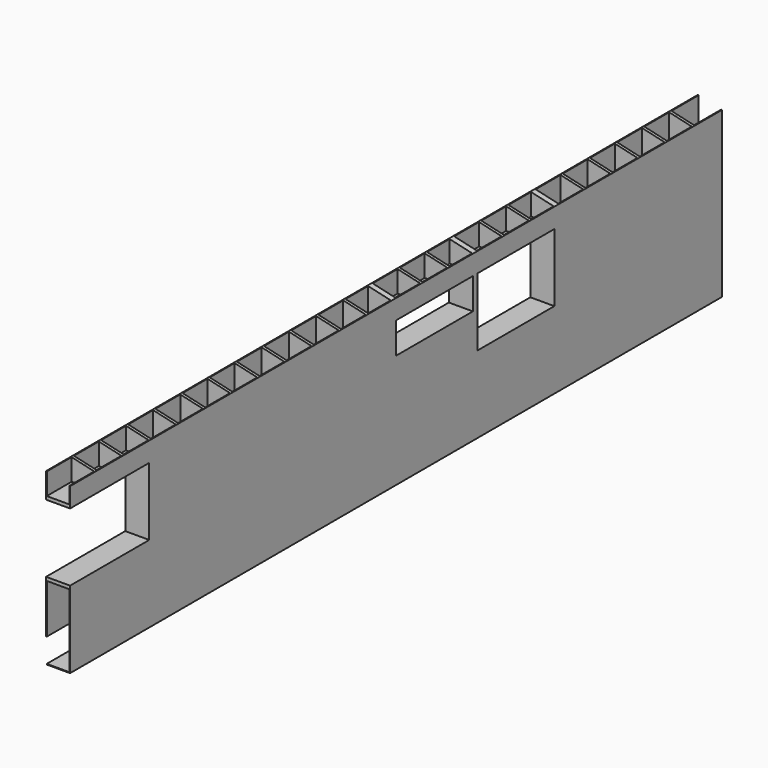
from build123d import *

# Parameters (mm, degrees)
F0_W     = 51
F0_H     = 590
F0_H_2   = 1290
F1_DEPTH = 400
F0_H_3   = 3200
F0_H_4   = 1940
F2_W     = 549
F2_H     = 590
F2_H_2   = 1290
F2_W_2   = 12600
F2_H_3   = 3200
F2_W_3   = 1698
F2_H_4   = 1200
F2_H_5   = 550
F3_DEPTH = 12
F4_W     = 12600
F4_H     = 2778
F4_W_2   = 1698
F4_H_2   = 1200
F4_H_3   = 550
F4_W_3   = 549
F4_H_4   = 590
F4_H_5   = 868
F5_DEPTH = 12
F7_DEPTH = 14400.001
F8_W     = 412
F8_H     = 14400
F9_DEPTH = 12


# Not quite as in the source:
# - a feature names something its author has since deleted; it is built from what else it names


with BuildPart() as f1:
    # F0 (on Right) → F1 (new body)
    with BuildSketch(Plane.YZ):
        with Locations((574.5, 2905)):
            Rectangle(F0_W, F0_H)
        with Locations((1174.5, 2905)):
            Rectangle(F0_W, F0_H)
        Polygon((1749, 2550), (1749, 1350), (1749, 1290), (1749, 0), (1800, 0), (1800, 3200), (1749, 3200), (1749, 2610), align=None)
        Polygon((0, 2610), (0, 2550), (1740, 2550), (1749, 2550), (1749, 2610), (1200, 2610), (1149, 2610), (600, 2610), (549, 2610), align=None)
        Polygon((0, 1350), (0, 1290), (549, 1290), (600, 1290), (1149, 1290), (1200, 1290), (1749, 1290), (1749, 1350), (1740, 1350), align=None)
        with Locations((1174.5, 645)):
            Rectangle(F0_W, F0_H_2)
        with Locations((574.5, 645)):
            Rectangle(F0_W, F0_H_2)
    extrude(amount=F1_DEPTH)



with BuildPart() as f1b:
    # F0 (on Right) → F1, piece 2 (new body)
    with BuildSketch(Plane.YZ):
        with Locations((2374.5, 1600)):
            Rectangle(F0_W, F0_H_3)
    extrude(amount=F1_DEPTH)


with BuildPart() as f1c:
    # F0 (on Right) → F1, piece 3 (new body)
    with BuildSketch(Plane.YZ):
        with Locations((2974.5, 1600)):
            Rectangle(F0_W, F0_H_3)
    extrude(amount=F1_DEPTH)


with BuildPart() as f1d:
    # F0 (on Right) → F1, piece 4 (new body)
    with BuildSketch(Plane.YZ):
        with Locations((3574.5, 1600)):
            Rectangle(F0_W, F0_H_3)
    extrude(amount=F1_DEPTH)


with BuildPart() as f1e:
    # F0 (on Right) → F1, piece 5 (new body)
    with BuildSketch(Plane.YZ):
        with Locations((4174.5, 1600)):
            Rectangle(F0_W, F0_H_3)
    extrude(amount=F1_DEPTH)


with BuildPart() as f1f:
    # F0 (on Right) → F1, piece 6 (new body)
    with BuildSketch(Plane.YZ):
        with Locations((4774.5, 1600)):
            Rectangle(F0_W, F0_H_3)
    extrude(amount=F1_DEPTH)


with BuildPart() as f1g:
    # F0 (on Right) → F1, piece 7 (new body)
    with BuildSketch(Plane.YZ):
        with Locations((5374.5, 1600)):
            Rectangle(F0_W, F0_H_3)
    extrude(amount=F1_DEPTH)


with BuildPart() as f1h:
    # F0 (on Right) → F1, piece 8 (new body)
    with BuildSketch(Plane.YZ):
        with Locations((5974.5, 1600)):
            Rectangle(F0_W, F0_H_3)
    extrude(amount=F1_DEPTH)


with BuildPart() as f1i:
    # F0 (on Right) → F1, piece 9 (new body)
    with BuildSketch(Plane.YZ):
        with Locations((6574.5, 1600)):
            Rectangle(F0_W, F0_H_3)
    extrude(amount=F1_DEPTH)


with BuildPart() as f1j:
    # F0 (on Right) → F1, piece 10 (new body)
    with BuildSketch(Plane.YZ):
        with Locations((7774.5, 2905)):
            Rectangle(F0_W, F0_H)
        with Locations((8374.5, 2905)):
            Rectangle(F0_W, F0_H)
        with Locations((9574.5, 2905)):
            Rectangle(F0_W, F0_H)
        with Locations((10174.5, 2905)):
            Rectangle(F0_W, F0_H)
        with Locations((10774.5, 1600)):
            Rectangle(F0_W, F0_H_3)
        Polygon((7149, 3200), (7149, 0), (7200, 0), (7200, 1940), (7749, 1940), (7800, 1940), (8349, 1940), (8400, 1940), (8898, 1940), (8898, 2000), (7200, 2000), (7200, 2550), (7200, 2610), (7200, 3200), align=None)
        with Locations((7774.5, 970)):
            Rectangle(F0_W, F0_H_4)
        Polygon((9549, 2610), (9000, 2610), (9000, 2550), (10698, 2550), (10698, 2610), (10200, 2610), (10149, 2610), (9600, 2610), align=None)
        Polygon((8949, 3200), (8949, 0), (9000, 0), (9000, 1290), (9000, 1350), (9000, 2550), (9000, 2610), (9000, 3200), align=None)
        with Locations((9574.5, 645)):
            Rectangle(F0_W, F0_H_2)
        with Locations((7123.5, 1600)):
            Rectangle(F0_W, F0_H_3)
        Polygon((7749, 2610), (7200, 2610), (7200, 2550), (8898, 2550), (8898, 2610), (8400, 2610), (8349, 2610), (7800, 2610), align=None)
        Polygon((9000, 1350), (9000, 1290), (9549, 1290), (9600, 1290), (10149, 1290), (10200, 1290), (10698, 1290), (10698, 1350), align=None)
        Polygon((8898, 2610), (8898, 2550), (8898, 2000), (8898, 1940), (8898, 0), (8949, 0), (8949, 3200), (8898, 3200), align=None)
        with Locations((10174.5, 645)):
            Rectangle(F0_W, F0_H_2)
        Polygon((10698, 2550), (10698, 1350), (10698, 1290), (10698, 0), (10749, 0), (10749, 3200), (10698, 3200), (10698, 2610), align=None)
        with Locations((8374.5, 970)):
            Rectangle(F0_W, F0_H_4)
    extrude(amount=F1_DEPTH)


with BuildPart() as f1k:
    # F0 (on Right) → F1, piece 11 (new body)
    with BuildSketch(Plane.YZ):
        with Locations((11374.5, 1600)):
            Rectangle(F0_W, F0_H_3)
    extrude(amount=F1_DEPTH)


with BuildPart() as f1l:
    # F0 (on Right) → F1, piece 12 (new body)
    with BuildSketch(Plane.YZ):
        with Locations((11974.5, 1600)):
            Rectangle(F0_W, F0_H_3)
    extrude(amount=F1_DEPTH)


with BuildPart() as f1m:
    # F0 (on Right) → F1, piece 13 (new body)
    with BuildSketch(Plane.YZ):
        with Locations((12574.5, 1600)):
            Rectangle(F0_W, F0_H_3)
    extrude(amount=F1_DEPTH)


with BuildPart() as f1n:
    # F0 (on Right) → F1, piece 14 (new body)
    with BuildSketch(Plane.YZ):
        with Locations((13174.5, 1600)):
            Rectangle(F0_W, F0_H_3)
    extrude(amount=F1_DEPTH)


with BuildPart() as f1o:
    # F0 (on Right) → F1, piece 15 (new body)
    with BuildSketch(Plane.YZ):
        with Locations((13774.5, 1600)):
            Rectangle(F0_W, F0_H_3)
    extrude(amount=F1_DEPTH)


with BuildPart() as f1_1:
    add(f1.part)

    add(f1b.part)  # F3 merges F1b

    add(f1c.part)  # F3 merges F1c

    add(f1d.part)  # F3 merges F1d

    add(f1e.part)  # F3 merges F1e

    add(f1f.part)  # F3 merges F1f

    add(f1g.part)  # F3 merges F1g

    add(f1h.part)  # F3 merges F1h

    add(f1i.part)  # F3 merges F1i

    add(f1j.part)  # F3 merges F1j

    add(f1k.part)  # F3 merges F1k

    add(f1l.part)  # F3 merges F1l

    add(f1m.part)  # F3 merges F1m

    add(f1n.part)  # F3 merges F1n

    add(f1o.part)  # F3 merges F1o
    # F2 (on face) → F3 (join)
    with BuildSketch(Plane.YZ.offset(400)):
        with Locations((274.5, 2905)):
            Rectangle(F2_W, F2_H)
        Polygon((600, 3200), (549, 3200), (549, 2610), (0, 2610), (0, 2550), (1749, 2550), (1749, 1350), (0, 1350), (0, 1290), (549, 1290), (549, 0), (600, 0), (600, 1290), (1149, 1290), (1149, 0), (1200, 0), (1200, 1290), (1749, 1290), (1749, 0), (1800, 0), (1800, 3200), (1749, 3200), (1749, 2610), (1200, 2610), (1200, 3200), (1149, 3200), (1149, 2610), (600, 2610), align=None)
        with Locations((874.5, 2905)):
            Rectangle(F2_W, F2_H)
        with Locations((1474.5, 2905)):
            Rectangle(F2_W, F2_H)
        with Locations((274.5, 645)):
            Rectangle(F2_W, F2_H_2)
        with Locations((8100, 1600)):
            Rectangle(F2_W_2, F2_H_3)
        with Locations((9849, 1950)):
            Rectangle(F2_W_3, F2_H_4, mode=Mode.SUBTRACT)
        with Locations((8049, 2275)):
            Rectangle(F2_W_3, F2_H_5, mode=Mode.SUBTRACT)
        with Locations((874.5, 645)):
            Rectangle(F2_W, F2_H_2)
        with Locations((1474.5, 645)):
            Rectangle(F2_W, F2_H_2)
    extrude(amount=F3_DEPTH)

    # F4 (on face) → F5 (join)
    with BuildSketch(Plane(origin=(0, 0, 0), x_dir=(0, -1, 0), z_dir=(-1, 0, 0))):
        with Locations((-8100, 1811)):
            Rectangle(F4_W, F4_H)
        with Locations((-9849, 1950)):
            Rectangle(F4_W_2, F4_H_2, mode=Mode.SUBTRACT)
        with Locations((-8049, 2275)):
            Rectangle(F4_W_2, F4_H_3, mode=Mode.SUBTRACT)
        Polygon((-1749, 3200), (-1800, 3200), (-1800, 422), (-1749, 422), (-1749, 1290), (-1200, 1290), (-1200, 422), (-1149, 422), (-1149, 1290), (-600, 1290), (-600, 422), (-549, 422), (-549, 1290), (0, 1290), (0, 1350), (-1749, 1350), (-1749, 2550), (0, 2550), (0, 2610), (-549, 2610), (-549, 3200), (-600, 3200), (-600, 2610), (-1149, 2610), (-1149, 3200), (-1200, 3200), (-1200, 2610), (-1749, 2610), align=None)
        with Locations((-1474.5, 2905)):
            Rectangle(F4_W_3, F4_H_4)
        with Locations((-1474.5, 856)):
            Rectangle(F4_W_3, F4_H_5)
        with Locations((-874.5, 2905)):
            Rectangle(F4_W_3, F4_H_4)
        with Locations((-874.5, 856)):
            Rectangle(F4_W_3, F4_H_5)
        with Locations((-274.5, 2905)):
            Rectangle(F4_W_3, F4_H_4)
        with Locations((-274.5, 856)):
            Rectangle(F4_W_3, F4_H_5)
    extrude(amount=F5_DEPTH)

    # F6 (on face) → F7 (cut, through all)
    with BuildSketch(Plane(origin=(0, 14400, 0), x_dir=(-1, 0, 0), z_dir=(0, 1, 0))):
        Polygon((-400, 3200), (-400, 2900), (12, 2995.1176947437), (12, 3245.1176947437), (-422, 3245.1176947437), (-422, 2894.9208997952), (-412, 2897.2295817065), (-412, 3200), align=None)
        Polygon((-412, 2897.2295817065), (-400, 2900), (-400, 3200), (-412, 3200), align=None)
        Polygon((-452, 2887.9948540615), (-422, 2894.9208997952), (-422, 3245.1176947437), (-452, 3245.1176947437), align=None)
    extrude(amount=-F7_DEPTH, mode=Mode.SUBTRACT)

    # F8 (on face) → F9 (join)
    with BuildSketch(Plane(origin=(0, 0, 0), x_dir=(1, 0, 0), z_dir=(0, 0, -1))):
        with Locations((206, -7200)):
            Rectangle(F8_W, F8_H)
    extrude(amount=F9_DEPTH)


solid = f1_1.part
